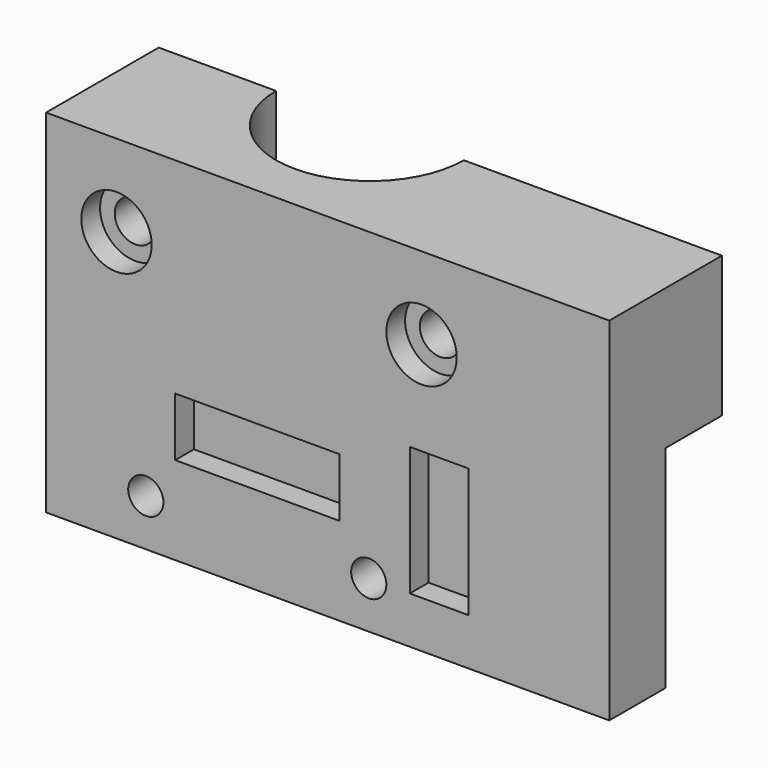
from build123d import *
from build123d import SkipClean  # not in build123d's __all__

# Parameters (mm, degrees)
F0_W     = 48
F0_H     = 30
F0_R     = 1.5
F0_W_2   = 14
F0_H_2   = 5
F0_W_3   = 5
F0_H_3   = 11
F0_R_2   = 3
F0_R_3   = 1.75
F1_DEPTH = 6
F2_DEPTH = 2
F5_DEPTH = 12
F6_DEPTH = 12.001
F7_DEPTH = 30.001


with BuildPart() as f1:
    # F0 (on Front) → F1 (new body)
    with BuildSketch(Plane.XZ):
        Rectangle(F0_W, F0_H)
        with Locations((-15.5, -11)):
            Circle(F0_R, mode=Mode.SUBTRACT)
        with Locations((-6, -5)):
            Rectangle(F0_W_2, F0_H_2, mode=Mode.SUBTRACT)
        with Locations((3.5, -11)):
            Circle(F0_R, mode=Mode.SUBTRACT)
        with Locations((9.5, -5.5)):
            Rectangle(F0_W_3, F0_H_3, mode=Mode.SUBTRACT)
        with Locations((-18, 8)):
            Circle(F0_R_2, mode=Mode.SUBTRACT)
        with Locations((8, 8)):
            Circle(F0_R_2, mode=Mode.SUBTRACT)
        with Locations((-6, -5)):
            Rectangle(F0_W_2, F0_H_2)
        with Locations((9.5, -5.5)):
            Rectangle(F0_W_3, F0_H_3)
        with Locations((8, 8)):
            Circle(F0_R_2)
        with Locations((8, 8)):
            Circle(F0_R_3, mode=Mode.SUBTRACT)
        with Locations((-18, 8)):
            Circle(F0_R_2)
        with Locations((-18, 8)):
            Circle(F0_R_3, mode=Mode.SUBTRACT)
    extrude(amount=-F1_DEPTH)

    # F0 (on Front) → F2 (cut)
    with BuildSketch(Plane.XZ):
        with Locations((9.5, -5.5)):
            Rectangle(F0_W_3, F0_H_3)
        with Locations((-6, -5)):
            Rectangle(F0_W_2, F0_H_2)
        with Locations((-18, 8)):
            Circle(F0_R_2)
        with Locations((-18, 8)):
            Circle(F0_R_3, mode=Mode.SUBTRACT)
        with Locations((8, 8)):
            Circle(F0_R_2)
        with Locations((8, 8)):
            Circle(F0_R_3, mode=Mode.SUBTRACT)
    extrude(amount=-F2_DEPTH, mode=Mode.SUBTRACT)

    # F4 (on face) → F5 (join)
    with BuildSketch(Plane.XY.offset(15)):
        with BuildLine():
            Line((-24, 12), (-24, 6))
            Line((-24, 6), (-11.2915026221, 6))
            ThreePointArc((-11.2915026221, 6), (-13.2915026221, 8.7084973779), (-14, 12))
            Line((-14, 12), (-24, 12))
        make_face()
        with BuildLine():
            ThreePointArc((2, 12), (1.2915026221, 8.7084973779), (-0.7084973779, 6))
            Line((-0.7084973779, 6), (24, 6))
            Line((24, 6), (24, 12))
            Line((24, 12), (2, 12))
        make_face()
    extrude(amount=-F5_DEPTH)

    # F0 (on Front) → F6 (cut, through all)
    with BuildSketch(Plane.XZ):
        with Locations((-18, 8)):
            Circle(F0_R_3)
        with Locations((8, 8)):
            Circle(F0_R_3)
    extrude(amount=-F6_DEPTH, mode=Mode.SUBTRACT)

    # F4 (on face) → F7 (cut, through all)
    with BuildSketch(Plane.XY.offset(15)):
        with BuildLine():
            Line((-0.7084973779, 6), (-11.2915026221, 6))
            ThreePointArc((-11.2915026221, 6), (-6, 4), (-0.7084973779, 6))
        make_face()
    with SkipClean():  # cleaning this boolean's faces spoils the solid; the shape is the same uncleaned
        extrude(amount=-F7_DEPTH, mode=Mode.SUBTRACT)


solid = f1.part
